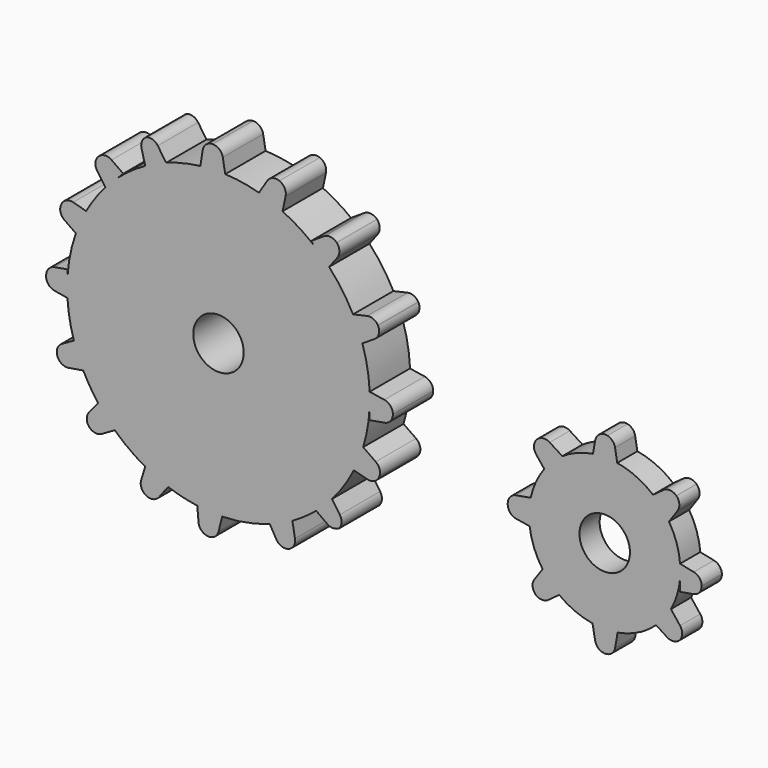
from build123d import *

# Parameters (mm, degrees)
F0_R     = 6.35
F1_DEPTH = 12.7
F2_R     = 6.35
F3_DEPTH = 6.35


# Not quite as in the source:
# - ends of sketch curves that miss each other by under 0.0002 mm in the source are joined
# - a feature of the source that left no trace in its solid (it failed there, or was rolled back) is left out


with BuildPart() as f1:
    # F0 (on Front) → F1 (new body)
    with BuildSketch(Plane.XZ):
        with BuildLine():
            ThreePointArc((-15.0035576595, 42.0839080108), (-14.9988274792, 42.430502183), (-14.9972507089, 42.7771250452))
            ThreePointArc((-14.9972507089, 42.7771250452), (-15.0062863673, 43.6068451943), (-15.0333890567, 44.4361717965))
            Line((-15.0333890567, 44.4361717965), (-15.0333890567, 41.1180782939))
            ThreePointArc((-15.0333890567, 41.1180782939), (-15.0154113194, 41.6008985757), (-15.0035576595, 42.0839080108))
        make_face()
        with BuildLine():
            ThreePointArc((-15.0333890567, 44.4361717965), (-15.0062863673, 43.6068451943), (-14.9972507089, 42.7771250452))
            ThreePointArc((-14.9972507089, 42.7771250452), (-14.9988274792, 42.430502183), (-15.0035576595, 42.0839080108))
            ThreePointArc((-15.0035576595, 42.0839080108), (-15.0154113194, 41.6008985757), (-15.0333890567, 41.1180782939))
            Line((-15.0333890567, 41.1180782939), (-15.0333890567, 38.1316341874))
            Line((-15.0333890567, 38.1316341874), (-11.2931131303, 38.7911457485))
            ThreePointArc((-11.2931131303, 38.7911457485), (-9.7793073012, 39.6708069424), (-9.1943390495, 41.3210263366))
            Line((-9.1943390495, 41.3210263366), (-9.194913427, 41.3722691845))
            ThreePointArc((-9.194913427, 41.3722691845), (-9.812979678, 43.0046386074), (-11.3385643935, 43.8527111865))
            Line((-11.3385643935, 43.8527111865), (-15.0333890567, 44.4361717965))
        make_face()
        with BuildLine():
            Line((-15.0333890567, 41.1180782939), (-15.0333890567, 44.4361717965))
            ThreePointArc((-15.0333890567, 44.4361717965), (-15.6058922132, 49.5600475823), (-16.8649366257, 54.5597145812))
            Line((-16.8649366257, 54.5597145812), (-19.2279926402, 60.2265765515))
            ThreePointArc((-19.2279926402, 60.2265765515), (-21.9425290756, 64.708684952), (-25.2463742538, 68.7759458008))
            Line((-25.2463742538, 68.7759458008), (-25.4824022418, 68.4632171136))
            Line((-25.4824022418, 68.4632171136), (-29.1813105141, 72.4358135631))
            ThreePointArc((-29.1813105141, 72.4358135631), (-32.9287932009, 75.1011613301), (-36.9700990178, 77.2955980464))
            Line((-36.9700990178, 77.2955980464), (-37.0124202716, 77.0978552404))
            Line((-37.0124202716, 77.0978552404), (-42.9074772554, 79.4892281853))
            ThreePointArc((-42.9074772554, 79.4892281853), (-47.1131650464, 80.4042524772), (-51.3952202234, 80.8390888966))
            Line((-51.3952202234, 80.8390888966), (-51.3535195971, 80.602592893))
            Line((-51.3535195971, 80.602592893), (-57.6627717197, 80.602592893))
            ThreePointArc((-57.6627717197, 80.602592893), (-62.0242551965, 79.816544464), (-66.2649555218, 78.529349451))
            Line((-66.2649555218, 78.529349451), (-71.5361466536, 76.118047593))
            ThreePointArc((-71.5361466536, 76.118047593), (-75.1123755418, 73.8728527035), (-78.4181898076, 71.245704974))
            Line((-78.4181898076, 71.245704974), (-81.5658306377, 68.0980641439))
            ThreePointArc((-81.5658306377, 68.0980641439), (-84.1757650921, 64.8165429989), (-86.409314292, 61.2681071672))
            Line((-86.409314292, 61.2681071672), (-86.3294839087, 61.2467166804))
            Line((-86.3294839087, 61.2467166804), (-89.0132026354, 55.4914632983))
            ThreePointArc((-89.0132026354, 55.4914632983), (-90.4329110895, 50.3704421035), (-91.1262707929, 45.1016962856))
            Line((-91.1262707929, 45.1016962856), (-91.1262707929, 40.4525538049))
            ThreePointArc((-91.1262707929, 40.4525538049), (-90.5811375904, 35.9530335849), (-89.5055410015, 31.5500863451))
            Line((-89.5055410015, 31.5500863451), (-89.2668263665, 31.684805394))
            Line((-89.2668263665, 31.684805394), (-87.15235036, 25.6932089908))
            ThreePointArc((-87.15235036, 25.6932089908), (-85.4075271484, 22.5866313315), (-83.3801304626, 19.6566321044))
            Line((-83.3801304626, 19.6566321044), (-83.2353912686, 19.8291255588))
            Line((-83.2353912686, 19.8291255588), (-79.2147433468, 15.0375039536))
            ThreePointArc((-79.2147433468, 15.0375039536), (-75.5557457853, 12.0000881686), (-71.5468746683, 9.4421377832))
            Line((-71.5468746683, 9.4421377832), (-71.4485760741, 9.7601605837))
            Line((-71.4485760741, 9.7601605837), (-65.7806115977, 6.8502220815))
            ThreePointArc((-65.7806115977, 6.8502220815), (-62.1516314122, 5.7686369637), (-58.4332100583, 5.0526298488))
            Line((-58.4332100583, 5.0526298488), (-58.4493496312, 5.2371060108))
            Line((-58.4493496312, 5.2371060108), (-52.1760489891, 4.6882633217))
            ThreePointArc((-52.1760489891, 4.6882633217), (-46.0933324969, 5.3264223859), (-40.1911006912, 6.9296524464))
            Line((-40.1911006912, 6.9296524464), (-40.4409376528, 7.3623827575))
            Line((-40.4409376528, 7.3623827575), (-34.4977696295, 9.5255190152))
            ThreePointArc((-34.4977696295, 9.5255190152), (-31.4067817733, 11.454073512), (-28.5141316627, 13.669046133))
            Line((-28.5141316627, 13.669046133), (-24.5144362494, 17.5852073418))
            ThreePointArc((-24.5144362494, 17.5852073418), (-21.4990486258, 21.4894848492), (-19.013398411, 25.7506452995))
            Line((-19.013398411, 25.7506452995), (-19.3611265761, 25.8438187806))
            Line((-19.3611265761, 25.8438187806), (-16.6671419061, 31.621087549))
            ThreePointArc((-16.6671419061, 31.621087549), (-15.5488004501, 36.3177223514), (-15.0333890567, 41.1180782939))
        make_face()
        with Locations((-53.0972507089, 42.7771250452)):
            Circle(F0_R, mode=Mode.SUBTRACT)
        with BuildLine():
            Line((-19.2279926402, 60.2265765515), (-16.8649366257, 54.5597145812))
            ThreePointArc((-16.8649366257, 54.5597145812), (-17.9321268546, 57.4408239069), (-19.2279926402, 60.2265765515))
        make_face()
        with BuildLine():
            ThreePointArc((-19.2279926402, 60.2265765515), (-17.9321268546, 57.4408239069), (-16.8649366257, 54.5597145812))
            Line((-16.8649366257, 54.5597145812), (-13.8186872434, 56.5105640631))
            ThreePointArc((-13.8186872434, 56.5105640631), (-12.7314322549, 58.0058053081), (-12.9458634732, 59.8420757249))
            ThreePointArc((-12.9458634732, 59.8420757249), (-14.1237366017, 60.87552765), (-15.6839341972, 61.0211004891))
            Line((-15.6839341972, 61.0211004891), (-19.2279926402, 60.2265765515))
        make_face()
        with BuildLine():
            Line((-13.5181342935, 29.4161286808), (-16.6671419061, 31.621087549))
            ThreePointArc((-16.6671419061, 31.621087549), (-17.7182993313, 28.6371179936), (-19.013398411, 25.7506452995))
            Line((-19.013398411, 25.7506452995), (-15.6474854146, 24.8487516304))
            ThreePointArc((-15.6474854146, 24.8487516304), (-13.903750519, 25.0062334323), (-12.6761763854, 26.2546218538))
            Line((-12.6761763854, 26.2546218538), (-12.6611097872, 26.287901113))
            ThreePointArc((-12.6611097872, 26.287901113), (-12.5252895753, 28.0066221759), (-13.5181342935, 29.4161286808))
        make_face()
        with BuildLine():
            ThreePointArc((-19.013398411, 25.7506452995), (-17.7182993313, 28.6371179936), (-16.6671419061, 31.621087549))
            Line((-16.6671419061, 31.621087549), (-19.3611265761, 25.8438187806))
            Line((-19.3611265761, 25.8438187806), (-19.013398411, 25.7506452995))
        make_face()
        with BuildLine():
            Line((-25.4824022418, 68.4632171136), (-25.2463742538, 68.7759458008))
            ThreePointArc((-25.2463742538, 68.7759458008), (-27.1492356687, 70.6753421114), (-29.1813105141, 72.4358135631))
            Line((-29.1813105141, 72.4358135631), (-25.4824022418, 68.4632171136))
        make_face()
        with BuildLine():
            ThreePointArc((-29.1813105141, 72.4358135631), (-27.1492356687, 70.6753421114), (-25.2463742538, 68.7759458008))
            Line((-25.2463742538, 68.7759458008), (-23.1720165619, 71.5243959446))
            ThreePointArc((-23.1720165619, 71.5243959446), (-22.6629050182, 73.1879791463), (-23.3437634431, 74.7889586709))
            ThreePointArc((-23.3437634431, 74.7889586709), (-24.88123861, 75.5442249196), (-26.5486019268, 75.1515971508))
            Line((-26.5486019268, 75.1515971508), (-29.7670901734, 73.0649360023))
            Line((-29.7670901734, 73.0649360023), (-29.1813105141, 72.4358135631))
        make_face()
        with BuildLine():
            Line((-22.5630056805, 14.7347232638), (-24.5144362494, 17.5852073418))
            ThreePointArc((-24.5144362494, 17.5852073418), (-26.442266165, 15.5535727612), (-28.5141316627, 13.669046133))
            Line((-28.5141316627, 13.669046133), (-25.7243685921, 11.6714326545))
            ThreePointArc((-25.7243685921, 11.6714326545), (-24.1530727926, 11.1982759233), (-22.6204013894, 11.7845916676))
            ThreePointArc((-22.6204013894, 11.7845916676), (-22.1193899067, 13.2504684602), (-22.5630056805, 14.7347232638))
        make_face()
        with BuildLine():
            ThreePointArc((-28.5141316627, 13.669046133), (-26.442266165, 15.5535727612), (-24.5144362494, 17.5852073418))
            Line((-24.5144362494, 17.5852073418), (-28.5141316627, 13.669046133))
        make_face()
        with BuildLine():
            Line((-37.0124202716, 77.0978552404), (-36.9700990178, 77.2955980464))
            ThreePointArc((-36.9700990178, 77.2955980464), (-39.8931551108, 78.5159255208), (-42.9074772554, 79.4892281853))
            Line((-42.9074772554, 79.4892281853), (-37.0124202716, 77.0978552404))
        make_face()
        with BuildLine():
            ThreePointArc((-42.9074772554, 79.4892281853), (-39.8931551108, 78.5159255208), (-36.9700990178, 77.2955980464))
            Line((-36.9700990178, 77.2955980464), (-36.2005639215, 80.891191643))
            ThreePointArc((-36.2005639215, 80.891191643), (-36.446660924, 82.6246414316), (-37.7559570519, 83.7870336004))
            Line((-37.7559570519, 83.7870336004), (-37.7667413657, 83.7912682008))
            ThreePointArc((-37.7667413657, 83.7912682008), (-39.4901495492, 83.8393665913), (-40.8472544061, 82.7760154595))
            Line((-40.8472544061, 82.7760154595), (-42.9074772554, 79.4892281853))
        make_face()
        with BuildLine():
            Line((-33.8359436619, 5.7721174372), (-34.4977696295, 9.5255190152))
            ThreePointArc((-34.4977696295, 9.5255190152), (-37.2910548188, 8.1105103925), (-40.1911006912, 6.9296524464))
            Line((-40.1911006912, 6.9296524464), (-38.5352964524, 4.0617153774))
            ThreePointArc((-38.5352964524, 4.0617153774), (-37.1918203475, 2.9403825082), (-35.4419269941, 2.9541193251))
            Line((-35.4419269941, 2.9541193251), (-35.4401633204, 2.9547829823))
            ThreePointArc((-35.4401633204, 2.9547829823), (-34.1301016673, 4.074217282), (-33.8359436619, 5.7721174372))
        make_face()
        with BuildLine():
            ThreePointArc((-40.1911006912, 6.9296524464), (-37.2910548188, 8.1105103925), (-34.4977696295, 9.5255190152))
            Line((-34.4977696295, 9.5255190152), (-40.4409376528, 7.3623827575))
            Line((-40.4409376528, 7.3623827575), (-40.1911006912, 6.9296524464))
        make_face()
        with BuildLine():
            Line((-51.3535195971, 80.602592893), (-51.3952202234, 80.8390888966))
            ThreePointArc((-51.3952202234, 80.8390888966), (-54.5338707307, 80.85003041), (-57.6627717197, 80.602592893))
            Line((-57.6627717197, 80.602592893), (-51.3535195971, 80.602592893))
        make_face()
        with BuildLine():
            ThreePointArc((-57.6627717197, 80.602592893), (-54.5338707307, 80.85003041), (-51.3952202234, 80.8390888966))
            Line((-51.3952202234, 80.8390888966), (-52.0155182816, 84.3569739972))
            ThreePointArc((-52.0155182816, 84.3569739972), (-52.8951794755, 85.8707798263), (-54.5453988697, 86.455748078))
            Line((-54.5453988697, 86.455748078), (-54.5966417176, 86.4551737004))
            ThreePointArc((-54.5966417176, 86.4551737004), (-56.2290111406, 85.8371074495), (-57.0770837197, 84.311522734))
            Line((-57.0770837197, 84.311522734), (-57.6627717197, 80.602592893))
        make_face()
        with BuildLine():
            Line((-53.0739942536, 1.079730934), (-52.1760489891, 4.6882633217))
            ThreePointArc((-52.1760489891, 4.6882633217), (-55.3121348986, 4.7415589521), (-58.4332100583, 5.0526298488))
            Line((-58.4332100583, 5.0526298488), (-58.1202602456, 1.4755971218))
            ThreePointArc((-58.1202602456, 1.4755971218), (-57.3758832996, -0.1091157438), (-55.7829268309, -0.8356841117))
            Line((-55.7829268309, -0.8356841117), (-55.7318289172, -0.8395780283))
            ThreePointArc((-55.7318289172, -0.8395780283), (-54.0518031295, -0.3661340756), (-53.0739942536, 1.079730934))
        make_face()
        with BuildLine():
            ThreePointArc((-58.4332100583, 5.0526298488), (-55.3121348986, 4.7415589521), (-52.1760489891, 4.6882633217))
            Line((-52.1760489891, 4.6882633217), (-58.4493496312, 5.2371060108))
            Line((-58.4493496312, 5.2371060108), (-58.4332100583, 5.0526298488))
        make_face()
        with BuildLine():
            Line((-71.5361466536, 76.118047593), (-66.2649555218, 78.529349451))
            ThreePointArc((-66.2649555218, 78.529349451), (-68.9464745708, 77.4240888801), (-71.5361466536, 76.118047593))
        make_face()
        with BuildLine():
            ThreePointArc((-71.5361466536, 76.118047593), (-68.9464745708, 77.4240888801), (-66.2649555218, 78.529349451))
            Line((-66.2649555218, 78.529349451), (-68.3890757431, 81.6105437185))
            ThreePointArc((-68.3890757431, 81.6105437185), (-69.5906197372, 82.547977821), (-71.11243796, 82.6289714181))
            ThreePointArc((-71.11243796, 82.6289714181), (-72.3149311287, 81.4080050246), (-72.4682607336, 79.7011837724))
            Line((-72.4682607336, 79.7011837724), (-71.5361466536, 76.118047593))
        make_face()
        with BuildLine():
            Line((-68.0716939545, 3.8292066318), (-65.7806115977, 6.8502220815))
            ThreePointArc((-65.7806115977, 6.8502220815), (-68.7175961961, 8.0263724367), (-71.5468746683, 9.4421377832))
            Line((-71.5468746683, 9.4421377832), (-72.569365858, 6.1340995119))
            ThreePointArc((-72.569365858, 6.1340995119), (-72.4460629383, 4.3135669552), (-71.1340116027, 3.0454724426))
            Line((-71.1340116027, 3.0454724426), (-71.0868898863, 3.0254963786))
            ThreePointArc((-71.0868898863, 3.0254963786), (-69.4413195731, 2.9097350401), (-68.0716939545, 3.8292066318))
        make_face()
        with BuildLine():
            ThreePointArc((-71.5468746683, 9.4421377832), (-68.7175961961, 8.0263724367), (-65.7806115977, 6.8502220815))
            Line((-65.7806115977, 6.8502220815), (-71.4485760741, 9.7601605837))
            Line((-71.4485760741, 9.7601605837), (-71.5468746683, 9.4421377832))
        make_face()
        with BuildLine():
            Line((-81.5658306377, 68.0980641439), (-78.4181898076, 71.245704974))
            ThreePointArc((-78.4181898076, 71.245704974), (-80.0380190721, 69.7178934084), (-81.5658306377, 68.0980641439))
        make_face()
        with BuildLine():
            ThreePointArc((-81.5658306377, 68.0980641439), (-80.0380190721, 69.7178934084), (-78.4181898076, 71.245704974))
            Line((-78.4181898076, 71.245704974), (-77.0629927637, 72.6009020179))
            Line((-77.0629927637, 72.6009020179), (-80.0260980124, 74.6756906495))
            ThreePointArc((-80.0260980124, 74.6756906495), (-81.7185347749, 75.1240986213), (-83.2990511165, 74.3708523148))
            Line((-83.2990511165, 74.3708523148), (-83.3753298068, 74.2928442347))
            ThreePointArc((-83.3753298068, 74.2928442347), (-84.090796282, 72.7242279831), (-83.6399070435, 71.0601522286))
            Line((-83.6399070435, 71.0601522286), (-81.5658306377, 68.0980641439))
        make_face()
        with BuildLine():
            Line((-82.4994251025, 13.1410920577), (-79.2147433468, 15.0375039536))
            ThreePointArc((-79.2147433468, 15.0375039536), (-81.3918542173, 17.2619254123), (-83.3801304626, 19.6566321044))
            Line((-83.3801304626, 19.6566321044), (-85.6669744193, 16.9312776032))
            ThreePointArc((-85.6669744193, 16.9312776032), (-86.2549144565, 15.1197111518), (-85.4182721401, 13.4087242642))
            ThreePointArc((-85.4182721401, 13.4087242642), (-84.0013475442, 12.8114069374), (-82.4994251025, 13.1410920577))
        make_face()
        with BuildLine():
            ThreePointArc((-83.3801304626, 19.6566321044), (-81.3918542173, 17.2619254123), (-79.2147433468, 15.0375039536))
            Line((-79.2147433468, 15.0375039536), (-83.2353912686, 19.8291255588))
            Line((-83.2353912686, 19.8291255588), (-83.3801304626, 19.6566321044))
        make_face()
        with BuildLine():
            Line((-86.3294839087, 61.2467166804), (-86.409314292, 61.2681071672))
            ThreePointArc((-86.409314292, 61.2681071672), (-87.8315556026, 58.434010545), (-89.0132026354, 55.4914632983))
            Line((-89.0132026354, 55.4914632983), (-86.3294839087, 61.2467166804))
        make_face()
        with BuildLine():
            ThreePointArc((-89.0132026354, 55.4914632983), (-87.8315556026, 58.434010545), (-86.409314292, 61.2681071672))
            Line((-86.409314292, 61.2681071672), (-89.7068377458, 62.1516759136))
            ThreePointArc((-89.7068377458, 62.1516759136), (-91.4505726415, 61.9941941118), (-92.678146775, 60.7458056902))
            Line((-92.678146775, 60.7458056902), (-92.7331441427, 60.6243269315))
            ThreePointArc((-92.7331441427, 60.6243269315), (-92.8689643546, 58.9056058686), (-91.8761196364, 57.4960993637))
            Line((-91.8761196364, 57.4960993637), (-89.0132026354, 55.4914632983))
        make_face()
        with BuildLine():
            Line((-90.836292926, 25.0808065088), (-87.15235036, 25.6932089908))
            ThreePointArc((-87.15235036, 25.6932089908), (-88.4504412817, 28.5728328655), (-89.5055410015, 31.5500863451))
            Line((-89.5055410015, 31.5500863451), (-92.5242530632, 29.8464705705))
            ThreePointArc((-92.5242530632, 29.8464705705), (-93.6990014082, 28.3960494525), (-93.565304519, 26.5343619826))
            Line((-93.565304519, 26.5343619826), (-93.5422410618, 26.4863626896))
            ThreePointArc((-93.5422410618, 26.4863626896), (-92.4236435969, 25.3323675361), (-90.836292926, 25.0808065088))
        make_face()
        with BuildLine():
            ThreePointArc((-89.5055410015, 31.5500863451), (-88.4504412817, 28.5728328655), (-87.15235036, 25.6932089908))
            Line((-87.15235036, 25.6932089908), (-89.2668263665, 31.684805394))
            Line((-89.2668263665, 31.684805394), (-89.5055410015, 31.5500863451))
        make_face()
        with BuildLine():
            Line((-91.1262707929, 40.4525538049), (-91.1262707929, 45.1016962856))
            ThreePointArc((-91.1262707929, 45.1016962856), (-91.1972507089, 42.7771250452), (-91.1262707929, 40.4525538049))
        make_face()
        with BuildLine():
            ThreePointArc((-91.1262707929, 40.4525538049), (-91.1972507089, 42.7771250452), (-91.1262707929, 45.1016962856))
            Line((-91.1262707929, 45.1016962856), (-91.1262707929, 46.8106707726))
            Line((-91.1262707929, 46.8106707726), (-94.3883187049, 46.2354837134))
            ThreePointArc((-94.3883187049, 46.2354837134), (-95.8143082629, 45.4561934325), (-96.4760829819, 43.9720122499))
            Line((-96.4760829819, 43.9720122499), (-96.4950493935, 43.770437076))
            ThreePointArc((-96.4950493935, 43.770437076), (-95.986388123, 41.9928489373), (-94.4072851166, 41.0310851542))
            Line((-94.4072851166, 41.0310851542), (-91.1262707929, 40.4525538049))
        make_face()
    extrude(amount=F1_DEPTH)


with BuildPart() as f1b:
    # F0 (on Front) → F1, piece 2 (new body)
    with BuildSketch(Plane.XZ):
        with BuildLine():
            ThreePointArc((-22.4007836708, 11.9906758782), (-22.5075354058, 11.8843758879), (-22.6204013894, 11.7845916676))
            ThreePointArc((-22.6204013894, 11.7845916676), (-22.7138208542, 11.6664035782), (-22.8140828063, 11.5539617628))
            Line((-22.8140828063, 11.5539617628), (-22.4007836708, 11.9906758782))
        make_face()
    extrude(amount=F1_DEPTH)


with BuildPart() as f1c:
    # F0 (on Front) → F1, piece 3 (new body)
    with BuildSketch(Plane.XZ):
        with BuildLine():
            ThreePointArc((-85.3943034089, 13.3874725262), (-85.406321277, 13.3980606094), (-85.4182721401, 13.4087242642))
            ThreePointArc((-85.4182721401, 13.4087242642), (-85.4304225822, 13.4191599443), (-85.4425069776, 13.429672035))
            Line((-85.4425069776, 13.429672035), (-85.3943034089, 13.3874725262))
        make_face()
    extrude(amount=F1_DEPTH)


with BuildPart() as f1d:
    # F0 (on Front) → F1, piece 4 (new body)
    with BuildSketch(Plane.XZ):
        with BuildLine():
            ThreePointArc((-71.3517940873, 82.5547019483), (-71.2330325738, 82.5947905468), (-71.11243796, 82.6289714181))
            ThreePointArc((-71.11243796, 82.6289714181), (-70.9982051277, 82.6805684418), (-70.8815659308, 82.7264671407))
            Line((-70.8815659308, 82.7264671407), (-71.3517940873, 82.5547019483))
        make_face()
    extrude(amount=F1_DEPTH)


with BuildPart() as f1e:
    # F0 (on Front) → F1, piece 5 (new body)
    with BuildSketch(Plane.XZ):
        with BuildLine():
            ThreePointArc((-23.3599696303, 74.8061366529), (-23.3518465721, 74.7975664971), (-23.3437634431, 74.7889586709))
            ThreePointArc((-23.3437634431, 74.7889586709), (-23.335561054, 74.7804644105), (-23.3273982422, 74.7719321102))
            Line((-23.3273982422, 74.7719321102), (-23.3599696303, 74.8061366529))
        make_face()
    extrude(amount=F1_DEPTH)


with BuildPart() as f1f:
    # F0 (on Front) → F1, piece 6 (new body)
    with BuildSketch(Plane.XZ):
        with BuildLine():
            ThreePointArc((-12.9753225797, 59.8958969168), (-12.960430508, 59.8690752755), (-12.9458634732, 59.8420757249))
            ThreePointArc((-12.9458634732, 59.8420757249), (-12.9303278925, 59.8156216142), (-12.9151129565, 59.7889817951))
            Line((-12.9151129565, 59.7889817951), (-12.9753225797, 59.8958969168))
        make_face()
    extrude(amount=F1_DEPTH)


with BuildPart() as f3:
    # F2 (on Front) → F3 (new body)
    with BuildSketch(Plane.XZ):
        with BuildLine():
            ThreePointArc((58.0384332363, 24.3035947121), (58.0888671822, 25.1025595433), (58.1056883996, 25.9029378482))
            ThreePointArc((58.1056883996, 25.9029378482), (58.0888671822, 26.7033161532), (58.0384332363, 27.5022809844))
            Line((58.0384332363, 27.5022809844), (58.0384332363, 24.3035947121))
        make_face()
        with BuildLine():
            ThreePointArc((58.0384332363, 27.5022809844), (58.0888671822, 26.7033161532), (58.1056883996, 25.9029378482))
            ThreePointArc((58.1056883996, 25.9029378482), (58.0888671822, 25.1025595433), (58.0384332363, 24.3035947121))
            Line((58.0384332363, 24.3035947121), (58.0384332363, 21.2614618056))
            Line((58.0384332363, 21.2614618056), (61.3884770837, 21.8521649225))
            ThreePointArc((61.3884770837, 21.8521649225), (62.8928910672, 22.7205713521), (63.4874105709, 24.3527287343))
            ThreePointArc((63.4874105709, 24.3527287343), (62.901928937, 25.9179154337), (61.4707115567, 26.780594376))
            Line((61.4707115567, 26.780594376), (58.0384332363, 27.5022809844))
        make_face()
        with BuildLine():
            Line((58.0384332363, 24.3035947121), (58.0384332363, 27.5022809844))
            ThreePointArc((58.0384332363, 27.5022809844), (57.1415497386, 31.886592219), (55.2466074246, 35.9406986109))
            Line((55.2466074246, 35.9406986109), (55.2046701154, 35.8808059264))
            Line((55.2046701154, 35.8808059264), (51.2214699402, 40.5622781986))
            ThreePointArc((51.2214699402, 40.5622781986), (46.987545795, 43.2231035016), (42.2070702798, 44.6904680809))
            Line((42.2070702798, 44.6904680809), (36.0870863624, 44.720214536))
            ThreePointArc((36.0870863624, 44.720214536), (32.0727706033, 43.6269712224), (28.3915296845, 41.6883177581))
            Line((28.3915296845, 41.6883177581), (28.4128618379, 41.6747575365))
            Line((28.4128618379, 41.6747575365), (23.8420316539, 37.3679781195))
            ThreePointArc((23.8420316539, 37.3679781195), (21.7251716384, 33.8121532827), (20.4261204482, 29.8831009032))
            Line((20.4261204482, 29.8831009032), (20.4876114346, 29.8939434232))
            Line((20.4876114346, 29.8939434232), (20.4876114346, 23.453107463))
            Line((20.4876114346, 23.453107463), (20.15717595, 23.5052875005))
            ThreePointArc((20.15717595, 23.5052875005), (21.2718030448, 19.0738880105), (23.4096308674, 15.0353997784))
            Line((23.4096308674, 15.0353997784), (23.5287070392, 15.2054581757))
            Line((23.5287070392, 15.2054581757), (27.6007837162, 10.6816481955))
            ThreePointArc((27.6007837162, 10.6816481955), (31.5783781494, 8.3817412161), (35.9909440212, 7.1010804428))
            Line((35.9909440212, 7.1010804428), (42.3030581897, 7.1317607555))
            ThreePointArc((42.3030581897, 7.1317607555), (47.4995569919, 8.8265335664), (52.0009164908, 11.9271169539))
            Line((52.0009164908, 11.9271169539), (51.5670618433, 12.207528677))
            Line((51.5670618433, 12.207528677), (55.7310194246, 16.6923007797))
            ThreePointArc((55.7310194246, 16.6923007797), (57.2863642612, 20.3761885658), (58.0384332363, 24.3035947121))
        make_face()
        with Locations((39.0556883996, 25.9029378482)):
            Circle(F2_R, mode=Mode.SUBTRACT)
        with BuildLine():
            Line((55.2046701154, 35.8808059264), (55.2466074246, 35.9406986109))
            ThreePointArc((55.2466074246, 35.9406986109), (53.4211109904, 38.4144179281), (51.2214699402, 40.5622781986))
            Line((51.2214699402, 40.5622781986), (55.2046701154, 35.8808059264))
        make_face()
        with BuildLine():
            ThreePointArc((51.2214699402, 40.5622781986), (53.4211109904, 38.4144179281), (55.2466074246, 35.9406986109))
            Line((55.2466074246, 35.9406986109), (57.3881044848, 38.9990733688))
            ThreePointArc((57.3881044848, 38.9990733688), (57.8376747078, 40.6786790706), (57.1015977002, 42.2539185248))
            ThreePointArc((57.1015977002, 42.2539185248), (55.5159617883, 42.9541214148), (53.8503845064, 42.474144696))
            Line((53.8503845064, 42.474144696), (51.2214699402, 40.5622781986))
        make_face()
        with BuildLine():
            Line((58.0281031875, 13.768054231), (55.7310194246, 16.6923007797))
            ThreePointArc((55.7310194246, 16.6923007797), (54.0563925434, 14.1606478165), (52.0009164908, 11.9271169539))
            Line((52.0009164908, 11.9271169539), (54.7365413697, 10.1590103068))
            ThreePointArc((54.7365413697, 10.1590103068), (56.413200096, 9.7697609069), (57.9530564848, 10.5388785065))
            ThreePointArc((57.9530564848, 10.5388785065), (58.5699902615, 12.1400007522), (58.0281031875, 13.768054231))
        make_face()
        with BuildLine():
            ThreePointArc((52.0009164908, 11.9271169539), (54.0563925434, 14.1606478165), (55.7310194246, 16.6923007797))
            Line((55.7310194246, 16.6923007797), (51.5670618433, 12.207528677))
            Line((51.5670618433, 12.207528677), (52.0009164908, 11.9271169539))
        make_face()
        with BuildLine():
            Line((36.0870863624, 44.720214536), (42.2070702798, 44.6904680809))
            ThreePointArc((42.2070702798, 44.6904680809), (39.1482806814, 44.9527128251), (36.0870863624, 44.720214536))
        make_face()
        with BuildLine():
            ThreePointArc((36.0870863624, 44.720214536), (39.1482806814, 44.9527128251), (42.2070702798, 44.6904680809))
            Line((42.2070702798, 44.6904680809), (41.6570861998, 47.9007490771))
            ThreePointArc((41.6570861998, 47.9007490771), (41.0037592823, 49.2120653973), (39.7348885761, 49.9444271135))
            Line((39.7348885761, 49.9444271135), (39.7215123887, 49.9475338546))
            ThreePointArc((39.7215123887, 49.9475338546), (37.762982795, 49.5854922573), (36.6677065924, 47.9219946313))
            Line((36.6677065924, 47.9219946313), (36.0870863624, 44.720214536))
        make_face()
        with BuildLine():
            Line((41.6878682092, 3.5408700816), (42.3030581897, 7.1317607555))
            ThreePointArc((42.3030581897, 7.1317607555), (39.1482806814, 6.8531628713), (35.9909440212, 7.1010804428))
            Line((35.9909440212, 7.1010804428), (36.6402284461, 3.520657577))
            ThreePointArc((36.6402284461, 3.520657577), (37.4243435348, 2.1003901738), (38.908160636, 1.4444307399))
            Line((38.908160636, 1.4444307399), (38.9530361084, 1.4403270853))
            ThreePointArc((38.9530361084, 1.4403270853), (40.7315384102, 1.9553789386), (41.6878682092, 3.5408700816))
        make_face()
        with BuildLine():
            ThreePointArc((35.9909440212, 7.1010804428), (39.1482806814, 6.8531628713), (42.3030581897, 7.1317607555))
            Line((42.3030581897, 7.1317607555), (35.9909440212, 7.1010804428))
        make_face()
        with BuildLine():
            Line((28.4128618379, 41.6747575365), (28.3915296845, 41.6883177581))
            ThreePointArc((28.3915296845, 41.6883177581), (25.937698199, 39.7167292574), (23.8420316539, 37.3679781195))
            Line((23.8420316539, 37.3679781195), (28.4128618379, 41.6747575365))
        make_face()
        with BuildLine():
            ThreePointArc((23.8420316539, 37.3679781195), (25.937698199, 39.7167292574), (28.3915296845, 41.6883177581))
            Line((28.3915296845, 41.6883177581), (25.2002861268, 43.7168972938))
            ThreePointArc((25.2002861268, 43.7168972938), (23.4895289976, 44.0893512498), (21.9441922663, 43.266340745))
            Line((21.9441922663, 43.266340745), (21.8905971915, 43.2063994337))
            ThreePointArc((21.8905971915, 43.2063994337), (21.2450859623, 41.5846870435), (21.7985649382, 39.9293028444))
            Line((21.7985649382, 39.9293028444), (23.8420316539, 37.3679781195))
        make_face()
        with BuildLine():
            Line((24.8397623741, 8.6737076293), (27.6007837162, 10.6816481955))
            ThreePointArc((27.6007837162, 10.6816481955), (25.3314643245, 12.6912697652), (23.4096308674, 15.0353997784))
            Line((23.4096308674, 15.0353997784), (21.3533011438, 12.0986565824))
            ThreePointArc((21.3533011438, 12.0986565824), (20.9022221136, 10.4369129788), (21.6146096982, 8.8693135322))
            ThreePointArc((21.6146096982, 8.8693135322), (23.1920739822, 8.1925825768), (24.8397623741, 8.6737076293))
        make_face()
        with BuildLine():
            ThreePointArc((23.4096308674, 15.0353997784), (25.3314643245, 12.6912697652), (27.6007837162, 10.6816481955))
            Line((27.6007837162, 10.6816481955), (23.5287070392, 15.2054581757))
            Line((23.5287070392, 15.2054581757), (23.4096308674, 15.0353997784))
        make_face()
        with BuildLine():
            Line((20.4876114346, 29.8939434232), (20.4261204482, 29.8831009032))
            ThreePointArc((20.4261204482, 29.8831009032), (20.0226032425, 26.7055394947), (20.15717595, 23.5052875005))
            Line((20.15717595, 23.5052875005), (20.4876114346, 23.453107463))
            Line((20.4876114346, 23.453107463), (20.4876114346, 29.8939434232))
        make_face()
        with BuildLine():
            ThreePointArc((20.15717595, 23.5052875005), (20.0226032425, 26.7055394947), (20.4261204482, 29.8831009032))
            Line((20.4261204482, 29.8831009032), (16.7387421317, 29.2329166179))
            ThreePointArc((16.7387421317, 29.2329166179), (15.2249363026, 28.353255424), (14.6399680509, 26.7030360298))
            Line((14.6399680509, 26.7030360298), (14.6420406442, 26.5181304927))
            ThreePointArc((14.6420406442, 26.5181304927), (15.2601068952, 24.8857610697), (16.7856916107, 24.0376884907))
            Line((16.7856916107, 24.0376884907), (20.15717595, 23.5052875005))
        make_face()
    extrude(amount=F3_DEPTH)


with BuildPart() as f3b:
    # F2 (on Front) → F3, piece 2 (new body)
    with BuildSketch(Plane.XZ):
        with BuildLine():
            ThreePointArc((63.4872511645, 24.3820455106), (63.4873731656, 24.3673873524), (63.4874105709, 24.3527287343))
            ThreePointArc((63.4874105709, 24.3527287343), (63.4877017485, 24.3380729607), (63.4879083414, 24.3234157508))
            Line((63.4879083414, 24.3234157508), (63.4872511645, 24.3820455106))
        make_face()
    extrude(amount=F3_DEPTH)


with BuildPart() as f3c:
    # F2 (on Front) → F3, piece 3 (new body)
    with BuildSketch(Plane.XZ):
        with BuildLine():
            ThreePointArc((57.9959452307, 10.5849620685), (57.9746436349, 10.5617874086), (57.9530564848, 10.5388785065))
            ThreePointArc((57.9530564848, 10.5388785065), (57.9323357675, 10.5151830486), (57.9113229974, 10.4917461901))
            Line((57.9113229974, 10.4917461901), (57.9959452307, 10.5849620685))
        make_face()
    extrude(amount=F3_DEPTH)


with BuildPart() as f3d:
    # F2 (on Front) → F3, piece 4 (new body)
    with BuildSketch(Plane.XZ):
        with BuildLine():
            ThreePointArc((21.6581394785, 8.8257034783), (21.6362423429, 8.8473765032), (21.6146096982, 8.8693135322))
            ThreePointArc((21.6146096982, 8.8693135322), (21.5921932842, 8.8904490222), (21.5700348793, 8.9118548544))
            Line((21.5700348793, 8.9118548544), (21.6581394785, 8.8257034783))
        make_face()
    extrude(amount=F3_DEPTH)


with BuildPart() as f3e:
    # F2 (on Front) → F3, piece 5 (new body)
    with BuildSketch(Plane.XZ):
        with BuildLine():
            ThreePointArc((57.08326615, 42.272026473), (57.0924548873, 42.2629957446), (57.1015977002, 42.2539185248))
            ThreePointArc((57.1015977002, 42.2539185248), (57.110877576, 42.2449814753), (57.1201120013, 42.2359974709))
            Line((57.1201120013, 42.2359974709), (57.08326615, 42.272026473))
        make_face()
    extrude(amount=F3_DEPTH)


solid = Compound([f1.part, f1b.part, f1c.part, f1d.part, f1e.part, f1f.part, f3.part, f3b.part, f3c.part, f3d.part, f3e.part])
